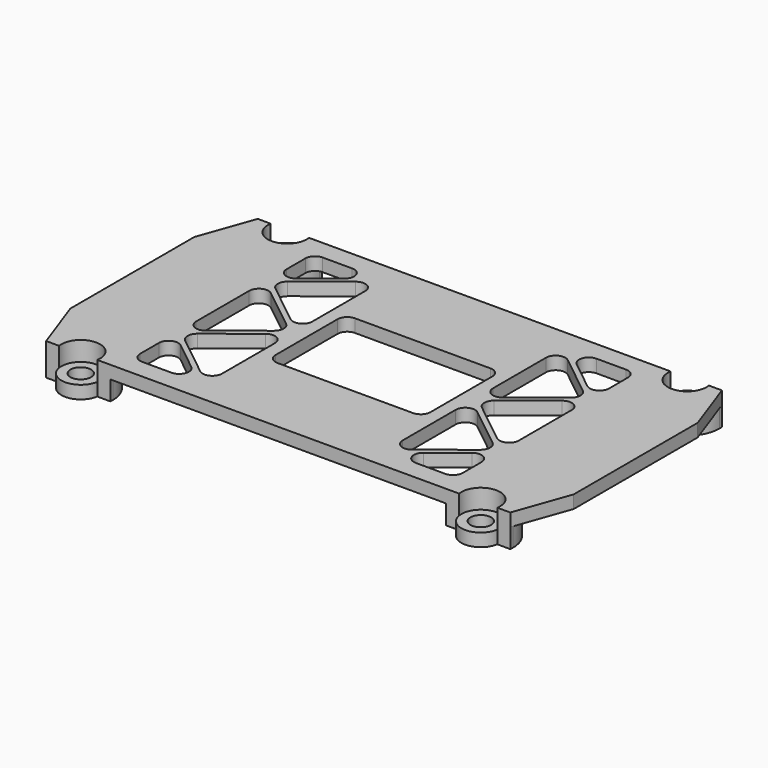
from build123d import *

# Parameters (mm, degrees)
F0_W     = 24
F0_H     = 15
F0_H_2   = 12
F0_W_2   = 12
F0_H_3   = 24
F1_DEPTH = 5
F2_DEPTH = 3
F3_R     = 1.6
F4_DEPTH = 3
F5_R     = 1.5


with BuildPart() as f1:
    # F0 (on Top) → F1 (new body)
    with BuildSketch(Plane.XY):
        with BuildLine():
            ThreePointArc((-29.4801315846, 20.5), (-29.4201599029, 20.2531901809), (-29.4, 20))
            ThreePointArc((-29.4, 20), (-31.2531901809, 18.4201599029), (-32.5198684154, 20.5))
            Line((-32.5198684154, 20.5), (-33.9580398915, 20.5))
            ThreePointArc((-33.9580398915, 20.5), (-31.2508787808, 17.0105084316), (-28, 20))
            ThreePointArc((-28, 20), (-28.0105084316, 20.2508787808), (-28.0419601085, 20.5))
            Line((-28.0419601085, 20.5), (-29.4801315846, 20.5))
        make_face()
        with BuildLine():
            ThreePointArc((-32.5198684154, 20.5), (-31, 21.6), (-29.4801315846, 20.5))
            Line((-29.4801315846, 20.5), (-28.0419601085, 20.5))
            ThreePointArc((-28.0419601085, 20.5), (-31, 23), (-33.9580398915, 20.5))
            Line((-33.9580398915, 20.5), (-32.5198684154, 20.5))
        make_face()
        with BuildLine():
            Line((-26.0250628145, 20.5), (-28.0419601085, 20.5))
            ThreePointArc((-28.0419601085, 20.5), (-28.0105084316, 20.2508787808), (-28, 20))
            ThreePointArc((-28, 20), (-31.2508787808, 17.0105084316), (-33.9580398915, 20.5))
            Line((-33.9580398915, 20.5), (-35.9749371855, 20.5))
            ThreePointArc((-35.9749371855, 20.5), (-31.2503138753, 15.0062696344), (-26, 20))
            ThreePointArc((-26, 20), (-26.0062696344, 20.2503138753), (-26.0250628145, 20.5))
        make_face()
        with BuildLine():
            Line((-12, 20.5), (-26.0250628145, 20.5))
            ThreePointArc((-26.0250628145, 20.5), (-26.0062696344, 20.2503138753), (-26, 20))
            ThreePointArc((-26, 20), (-31.2503138753, 15.0062696344), (-35.9749371855, 20.5))
            Line((-35.9749371855, 20.5), (-39, 12))
            Line((-39, 12), (-27, 12))
            Line((-27, 12), (-27, -12))
            Line((-27, -12), (-39, -12))
            Line((-39, -12), (-35.9749371855, -20.5))
            ThreePointArc((-35.9749371855, -20.5), (-31.2503138753, -15.0062696344), (-26, -20))
            ThreePointArc((-26, -20), (-26.0062696344, -20.2503138753), (-26.0250628145, -20.5))
            Line((-26.0250628145, -20.5), (-12, -20.5))
            Line((-12, -20.5), (-12, -8.5))
            Line((-12, -8.5), (12, -8.5))
            Line((12, -8.5), (12, -20.5))
            Line((12, -20.5), (26.0250628145, -20.5))
            ThreePointArc((26.0250628145, -20.5), (30.7496861247, -15.0062696344), (36, -20))
            ThreePointArc((36, -20), (35.9937303656, -20.2503138753), (35.9749371855, -20.5))
            Line((35.9749371855, -20.5), (39, -12))
            Line((39, -12), (27, -12))
            Line((27, -12), (27, 12))
            Line((27, 12), (39, 12))
            Line((39, 12), (35.9749371855, 20.5))
            ThreePointArc((35.9749371855, 20.5), (35.9937303656, 20.2503138753), (36, 20))
            ThreePointArc((36, 20), (30.7496861247, 15.0062696344), (26.0250628145, 20.5))
            Line((26.0250628145, 20.5), (12, 20.5))
            Line((12, 20.5), (12, 8.5))
            Line((12, 8.5), (-12, 8.5))
            Line((-12, 8.5), (-12, 20.5))
        make_face()
        Polygon((-14.6425459564, 17.5), (-14, 17.5), (-14, 16.9888838983), (-14, 0.5111161017), (-13.3574540436, 0), (-14, -0.5111161017), (-14, -16.9888838983), (-14, -17.5), (-14.6425459564, -17.5), (-25, -17.5), (-25, -9.2611161017), (-25.6425459564, -8.75), (-25, -8.2388838983), (-25, 8.2388838983), (-25.6425459564, 8.75), (-25, 9.2611161017), (-25, 17.5), align=None, mode=Mode.SUBTRACT)
        Rectangle(F0_W, F0_H, mode=Mode.SUBTRACT)
        Polygon((14, 16.9888838983), (14, 17.5), (14.6425459564, 17.5), (25, 17.5), (25, 9.2611161017), (25.6425459564, 8.75), (25, 8.2388838983), (25, -8.2388838983), (25.6425459564, -8.75), (25, -9.2611161017), (25, -17.5), (14.6425459564, -17.5), (14, -17.5), (14, -16.9888838983), (14, -0.5111161017), (13.3574540436, 0), (14, 0.5111161017), align=None, mode=Mode.SUBTRACT)
        with Locations((0, 14.5)):
            Rectangle(F0_W, F0_H_2)
        with Locations((-33, 0)):
            Rectangle(F0_W_2, F0_H_3)
        with BuildLine():
            Line((28.0419601085, 20.5), (26.0250628145, 20.5))
            ThreePointArc((26.0250628145, 20.5), (30.7496861247, 15.0062696344), (36, 20))
            ThreePointArc((36, 20), (35.9937303656, 20.2503138753), (35.9749371855, 20.5))
            Line((35.9749371855, 20.5), (33.9580398915, 20.5))
            ThreePointArc((33.9580398915, 20.5), (33.9894915684, 20.2508787808), (34, 20))
            ThreePointArc((34, 20), (30.7491212192, 17.0105084316), (28.0419601085, 20.5))
        make_face()
        with BuildLine():
            ThreePointArc((-26, -20), (-31.2503138753, -15.0062696344), (-35.9749371855, -20.5))
            Line((-35.9749371855, -20.5), (-33.9580398915, -20.5))
            ThreePointArc((-33.9580398915, -20.5), (-31.2508787808, -17.0105084316), (-28, -20))
            ThreePointArc((-28, -20), (-28.0105084316, -20.2508787808), (-28.0419601085, -20.5))
            Line((-28.0419601085, -20.5), (-26.0250628145, -20.5))
            ThreePointArc((-26.0250628145, -20.5), (-26.0062696344, -20.2503138753), (-26, -20))
        make_face()
        with BuildLine():
            ThreePointArc((33.9580398915, 20.5), (31, 23), (28.0419601085, 20.5))
            Line((28.0419601085, 20.5), (29.4801315846, 20.5))
            ThreePointArc((29.4801315846, 20.5), (31, 21.6), (32.5198684154, 20.5))
            Line((32.5198684154, 20.5), (33.9580398915, 20.5))
        make_face()
        with BuildLine():
            Line((29.4801315846, 20.5), (28.0419601085, 20.5))
            ThreePointArc((28.0419601085, 20.5), (30.7491212192, 17.0105084316), (34, 20))
            ThreePointArc((34, 20), (33.9894915684, 20.2508787808), (33.9580398915, 20.5))
            Line((33.9580398915, 20.5), (32.5198684154, 20.5))
            ThreePointArc((32.5198684154, 20.5), (32.5798400971, 20.2531901809), (32.6, 20))
            ThreePointArc((32.6, 20), (30.7468098191, 18.4201599029), (29.4801315846, 20.5))
        make_face()
        with BuildLine():
            ThreePointArc((-28, -20), (-31.2508787808, -17.0105084316), (-33.9580398915, -20.5))
            Line((-33.9580398915, -20.5), (-32.5198684154, -20.5))
            ThreePointArc((-32.5198684154, -20.5), (-31.2531901809, -18.4201599029), (-29.4, -20))
            ThreePointArc((-29.4, -20), (-29.4201599029, -20.2531901809), (-29.4801315846, -20.5))
            Line((-29.4801315846, -20.5), (-28.0419601085, -20.5))
            ThreePointArc((-28.0419601085, -20.5), (-28.0105084316, -20.2508787808), (-28, -20))
        make_face()
        with BuildLine():
            Line((-32.5198684154, -20.5), (-33.9580398915, -20.5))
            ThreePointArc((-33.9580398915, -20.5), (-31, -23), (-28.0419601085, -20.5))
            Line((-28.0419601085, -20.5), (-29.4801315846, -20.5))
            ThreePointArc((-29.4801315846, -20.5), (-31, -21.6), (-32.5198684154, -20.5))
        make_face()
        with Locations((33, 0)):
            Rectangle(F0_W_2, F0_H_3)
        with Locations((0, -14.5)):
            Rectangle(F0_W, F0_H_2)
        with BuildLine():
            Line((33.9580398915, -20.5), (35.9749371855, -20.5))
            ThreePointArc((35.9749371855, -20.5), (35.9937303656, -20.2503138753), (36, -20))
            ThreePointArc((36, -20), (30.7496861247, -15.0062696344), (26.0250628145, -20.5))
            Line((26.0250628145, -20.5), (28.0419601085, -20.5))
            ThreePointArc((28.0419601085, -20.5), (30.7491212192, -17.0105084316), (34, -20))
            ThreePointArc((34, -20), (33.9894915684, -20.2508787808), (33.9580398915, -20.5))
        make_face()
        with BuildLine():
            ThreePointArc((28.0419601085, -20.5), (31, -23), (33.9580398915, -20.5))
            Line((33.9580398915, -20.5), (32.5198684154, -20.5))
            ThreePointArc((32.5198684154, -20.5), (31, -21.6), (29.4801315846, -20.5))
            Line((29.4801315846, -20.5), (28.0419601085, -20.5))
        make_face()
        with BuildLine():
            Line((32.5198684154, -20.5), (33.9580398915, -20.5))
            ThreePointArc((33.9580398915, -20.5), (33.9894915684, -20.2508787808), (34, -20))
            ThreePointArc((34, -20), (30.7491212192, -17.0105084316), (28.0419601085, -20.5))
            Line((28.0419601085, -20.5), (29.4801315846, -20.5))
            ThreePointArc((29.4801315846, -20.5), (30.7468098191, -18.4201599029), (32.6, -20))
            ThreePointArc((32.6, -20), (32.5798400971, -20.2531901809), (32.5198684154, -20.5))
        make_face()
        Polygon((-25, 8.75), (-14, 17.5), (-14.6425459564, 17.5), (-25, 9.2611161017), align=None)
        Polygon((-14, 16.9888838983), (-14, 17.5), (-25, 8.75), (-14, 0), (-14, 0.5111161017), (-24.3574540436, 8.75), align=None)
        Polygon((-25, 8.2388838983), (-25, 8.75), (-25, 9.2611161017), (-25.6425459564, 8.75), align=None)
        Polygon((-14, 0), (-25, 8.75), (-25, 8.2388838983), (-14.6425459564, 0), (-25, -8.2388838983), (-25, -8.75), align=None)
        Polygon((-13.3574540436, 0), (-14, 0.5111161017), (-14, 0), (-14, -0.5111161017), align=None)
        Polygon((-14, -0.5111161017), (-14, 0), (-25, -8.75), (-14, -17.5), (-14, -16.9888838983), (-24.3574540436, -8.75), align=None)
        Polygon((-25, -8.75), (-25, -8.2388838983), (-25.6425459564, -8.75), (-25, -9.2611161017), align=None)
        Polygon((-14, -17.5), (-25, -8.75), (-25, -9.2611161017), (-14.6425459564, -17.5), align=None)
        Polygon((25, 8.75), (14, 17.5), (14, 16.9888838983), (24.3574540436, 8.75), (14, 0.5111161017), (14, 0), align=None)
        Polygon((14.6425459564, 17.5), (14, 17.5), (25, 8.75), (25, 9.2611161017), align=None)
        Polygon((25, 9.2611161017), (25, 8.75), (25, 8.2388838983), (25.6425459564, 8.75), align=None)
        Polygon((25, 8.2388838983), (25, 8.75), (14, 0), (25, -8.75), (25, -8.2388838983), (14.6425459564, 0), align=None)
        Polygon((14, 0), (14, 0.5111161017), (13.3574540436, 0), (14, -0.5111161017), align=None)
        Polygon((25, -8.75), (14, 0), (14, -0.5111161017), (24.3574540436, -8.75), (14, -16.9888838983), (14, -17.5), align=None)
        Polygon((25.6425459564, -8.75), (25, -8.2388838983), (25, -8.75), (25, -9.2611161017), align=None)
        Polygon((25, -9.2611161017), (25, -8.75), (14, -17.5), (14.6425459564, -17.5), align=None)
    extrude(amount=F1_DEPTH)

    # F0 (on Top) → F2 (cut)
    with BuildSketch(Plane.XY):
        with Locations((-33, 0)):
            Rectangle(F0_W_2, F0_H_3)
        with BuildLine():
            Line((-12, 20.5), (-26.0250628145, 20.5))
            ThreePointArc((-26.0250628145, 20.5), (-26.0062696344, 20.2503138753), (-26, 20))
            ThreePointArc((-26, 20), (-31.2503138753, 15.0062696344), (-35.9749371855, 20.5))
            Line((-35.9749371855, 20.5), (-39, 12))
            Line((-39, 12), (-27, 12))
            Line((-27, 12), (-27, -12))
            Line((-27, -12), (-39, -12))
            Line((-39, -12), (-35.9749371855, -20.5))
            ThreePointArc((-35.9749371855, -20.5), (-31.2503138753, -15.0062696344), (-26, -20))
            ThreePointArc((-26, -20), (-26.0062696344, -20.2503138753), (-26.0250628145, -20.5))
            Line((-26.0250628145, -20.5), (-12, -20.5))
            Line((-12, -20.5), (-12, -8.5))
            Line((-12, -8.5), (12, -8.5))
            Line((12, -8.5), (12, -20.5))
            Line((12, -20.5), (26.0250628145, -20.5))
            ThreePointArc((26.0250628145, -20.5), (30.7496861247, -15.0062696344), (36, -20))
            ThreePointArc((36, -20), (35.9937303656, -20.2503138753), (35.9749371855, -20.5))
            Line((35.9749371855, -20.5), (39, -12))
            Line((39, -12), (27, -12))
            Line((27, -12), (27, 12))
            Line((27, 12), (39, 12))
            Line((39, 12), (35.9749371855, 20.5))
            ThreePointArc((35.9749371855, 20.5), (35.9937303656, 20.2503138753), (36, 20))
            ThreePointArc((36, 20), (30.7496861247, 15.0062696344), (26.0250628145, 20.5))
            Line((26.0250628145, 20.5), (12, 20.5))
            Line((12, 20.5), (12, 8.5))
            Line((12, 8.5), (-12, 8.5))
            Line((-12, 8.5), (-12, 20.5))
        make_face()
        Polygon((-14.6425459564, 17.5), (-14, 17.5), (-14, 16.9888838983), (-14, 0.5111161017), (-13.3574540436, 0), (-14, -0.5111161017), (-14, -16.9888838983), (-14, -17.5), (-14.6425459564, -17.5), (-25, -17.5), (-25, -9.2611161017), (-25.6425459564, -8.75), (-25, -8.2388838983), (-25, 8.2388838983), (-25.6425459564, 8.75), (-25, 9.2611161017), (-25, 17.5), align=None, mode=Mode.SUBTRACT)
        Rectangle(F0_W, F0_H, mode=Mode.SUBTRACT)
        Polygon((14, 16.9888838983), (14, 17.5), (14.6425459564, 17.5), (25, 17.5), (25, 9.2611161017), (25.6425459564, 8.75), (25, 8.2388838983), (25, -8.2388838983), (25.6425459564, -8.75), (25, -9.2611161017), (25, -17.5), (14.6425459564, -17.5), (14, -17.5), (14, -16.9888838983), (14, -0.5111161017), (13.3574540436, 0), (14, 0.5111161017), align=None, mode=Mode.SUBTRACT)
        Polygon((-25, 8.2388838983), (-25, 8.75), (-25, 9.2611161017), (-25.6425459564, 8.75), align=None)
        Polygon((-25, -8.75), (-25, -8.2388838983), (-25.6425459564, -8.75), (-25, -9.2611161017), align=None)
        Polygon((-25, 8.75), (-14, 17.5), (-14.6425459564, 17.5), (-25, 9.2611161017), align=None)
        Polygon((-14, 16.9888838983), (-14, 17.5), (-25, 8.75), (-14, 0), (-14, 0.5111161017), (-24.3574540436, 8.75), align=None)
        Polygon((-14, -0.5111161017), (-14, 0), (-25, -8.75), (-14, -17.5), (-14, -16.9888838983), (-24.3574540436, -8.75), align=None)
        Polygon((-14, 0), (-25, 8.75), (-25, 8.2388838983), (-14.6425459564, 0), (-25, -8.2388838983), (-25, -8.75), align=None)
        Polygon((-13.3574540436, 0), (-14, 0.5111161017), (-14, 0), (-14, -0.5111161017), align=None)
        Polygon((-14, -17.5), (-25, -8.75), (-25, -9.2611161017), (-14.6425459564, -17.5), align=None)
        with Locations((0, 14.5)):
            Rectangle(F0_W, F0_H_2)
        with Locations((0, -14.5)):
            Rectangle(F0_W, F0_H_2)
        with Locations((33, 0)):
            Rectangle(F0_W_2, F0_H_3)
        Polygon((25, 9.2611161017), (25, 8.75), (25, 8.2388838983), (25.6425459564, 8.75), align=None)
        Polygon((25.6425459564, -8.75), (25, -8.2388838983), (25, -8.75), (25, -9.2611161017), align=None)
        Polygon((14.6425459564, 17.5), (14, 17.5), (25, 8.75), (25, 9.2611161017), align=None)
        Polygon((25, 8.75), (14, 17.5), (14, 16.9888838983), (24.3574540436, 8.75), (14, 0.5111161017), (14, 0), align=None)
        Polygon((14, 0), (14, 0.5111161017), (13.3574540436, 0), (14, -0.5111161017), align=None)
        Polygon((25, -8.75), (14, 0), (14, -0.5111161017), (24.3574540436, -8.75), (14, -16.9888838983), (14, -17.5), align=None)
        Polygon((25, -9.2611161017), (25, -8.75), (14, -17.5), (14.6425459564, -17.5), align=None)
        Polygon((25, 8.2388838983), (25, 8.75), (14, 0), (25, -8.75), (25, -8.2388838983), (14.6425459564, 0), align=None)
    extrude(amount=F2_DEPTH, mode=Mode.SUBTRACT)

    # F3 (on face) → F4 (cut)
    with BuildSketch(Plane.XY.offset(5)):
        with BuildLine():
            ThreePointArc((-28, 20), (-28.0105084316, 20.2508787808), (-28.0419601085, 20.5))
            ThreePointArc((-28.0419601085, 20.5), (-31, 23), (-33.9580398915, 20.5))
            ThreePointArc((-33.9580398915, 20.5), (-31.2508787808, 17.0105084316), (-28, 20))
        make_face()
        with Locations((-31, 20)):
            Circle(F3_R, mode=Mode.SUBTRACT)
        with BuildLine():
            ThreePointArc((-33.9580398915, -20.5), (-31, -23), (-28.0419601085, -20.5))
            ThreePointArc((-28.0419601085, -20.5), (-28.0105084316, -20.2508787808), (-28, -20))
            ThreePointArc((-28, -20), (-31.2508787808, -17.0105084316), (-33.9580398915, -20.5))
        make_face()
        with Locations((-31, -20)):
            Circle(F3_R, mode=Mode.SUBTRACT)
        with BuildLine():
            ThreePointArc((28.0419601085, -20.5), (31, -23), (33.9580398915, -20.5))
            ThreePointArc((33.9580398915, -20.5), (33.9894915684, -20.2508787808), (34, -20))
            ThreePointArc((34, -20), (30.7491212192, -17.0105084316), (28.0419601085, -20.5))
        make_face()
        with Locations((31, -20)):
            Circle(F3_R, mode=Mode.SUBTRACT)
        with BuildLine():
            ThreePointArc((28.0419601085, 20.5), (30.7491212192, 17.0105084316), (34, 20))
            ThreePointArc((34, 20), (33.9894915684, 20.2508787808), (33.9580398915, 20.5))
            ThreePointArc((33.9580398915, 20.5), (31, 23), (28.0419601085, 20.5))
        make_face()
        with Locations((31, 20)):
            Circle(F3_R, mode=Mode.SUBTRACT)
    extrude(amount=-F4_DEPTH, mode=Mode.SUBTRACT)

    # F5
    f5_edges = [f1.edges().sort_by_distance(p)[0] for p in [
        (25, -17.5, 4),
        (14.642546, -17.5, 4),
        (25, -9.261116, 4),
        (24.357454, -8.75, 4),
        (14, -16.988884, 4),
        (14, -0.511116, 4),
        (25, -8.238884, 4),
        (14.642546, 0, 4),
        (25, 8.238884, 4),
        (14, 0.511116, 4),
        (24.357454, 8.75, 4),
        (14, 16.988884, 4),
        (25, 9.261116, 4),
        (14.642546, 17.5, 4),
        (25, 17.5, 4),
        (-25, 17.5, 4),
        (-25, 8.238884, 4),
        (-25, -9.261116, 4),
        (-25, -17.5, 4),
        (-25, -8.238884, 4),
        (-25, 9.261116, 4),
        (-24.357454, 8.75, 4),
        (-24.357454, -8.75, 4),
        (-14.642546, 0, 4),
        (-14.642546, -17.5, 4),
        (-14.642546, 17.5, 4),
        (-14, 16.988884, 4),
        (-14, -0.511116, 4),
        (-14, 0.511116, 4),
        (-14, -16.988884, 4),
        (-12, -7.5, 4),
        (12, -7.5, 4),
        (12, 7.5, 4),
        (-12, 7.5, 4),
    ]]
    fillet(f5_edges, radius=F5_R)


solid = f1.part
